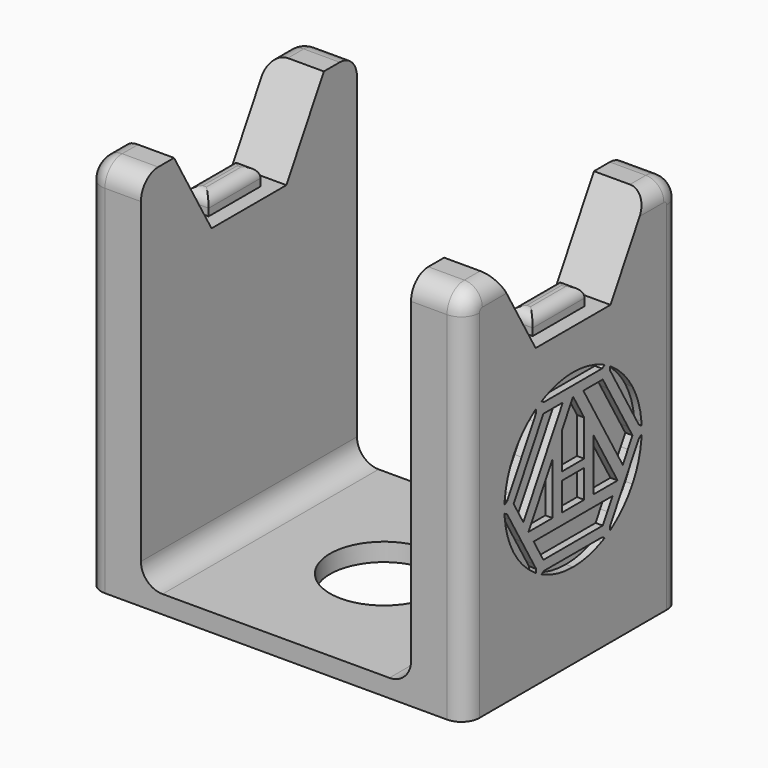
from build123d import *

# Parameters (mm, degrees)
F1_DEPTH  = 75
F3_DEPTH  = 122
F4_W      = 7
F4_H      = 18
F5_DEPTH  = 5
F6_R      = 3
F7_R      = 6
F8_R      = 5
F10_DEPTH = 2
F12_DEPTH = 2
F14_DEPTH = 25


with BuildPart() as f1:
    # F0 (on Front) → F1 (new body)
    with BuildSketch(Plane.XZ):
        Polygon((-52.5, -2.5), (52.5, -2.5), (52.5, 2.5), (37.5, 2.5), (0, 2.5), (-37.5, 2.5), (-52.5, 2.5), align=None)
        Polygon((37.5, 2.5), (52.5, 2.5), (52.5, 102.5), (37.5, 102.5), (37.5, 40), align=None)
        Polygon((-52.5, 102.5), (-52.5, 2.5), (-37.5, 2.5), (-37.5, 40), (-37.5, 102.5), align=None)
    extrude(amount=F1_DEPTH)

    # F2 (on face) → F3 (cut)
    with BuildSketch(Plane.YZ.offset(52.5)):
        Polygon((-24.5, 79.9833395016), (-11.5, 102.5), (-24.5, 125.0166604984), (-50.5, 125.0166604984), (-63.5, 102.5), (-50.5, 79.9833395016), align=None)
    extrude(amount=-F3_DEPTH, mode=Mode.SUBTRACT)

    # F4 (on face) → F5 (join)
    with BuildSketch(Plane.XY.offset(79.9833395016)):
        with Locations((45, -37.5)):
            Rectangle(F4_W, F4_H)
        with Locations((-45, -37.5)):
            Rectangle(F4_W, F4_H)
    extrude(amount=F5_DEPTH)

    # F6
    f6_edges = [f1.edges().sort_by_distance(p)[0] for p in [
        (-48.5, -37.5, 84.98334),
        (-45, -28.5, 84.98334),
        (-41.5, -37.5, 84.98334),
        (-45, -46.5, 84.98334),
        (41.5, -37.5, 84.98334),
        (45, -28.5, 84.98334),
        (48.5, -37.5, 84.98334),
        (45, -46.5, 84.98334),
    ]]
    fillet(f6_edges, radius=F6_R)

    # F7
    f7_edges = [f1.edges().sort_by_distance(p)[0] for p in [
        (-37.5, -37.5, 2.5),
        (37.5, -37.5, 2.5),
        (-45, -75, 102.5),
        (45, -75, 102.5),
        (45, 0, 102.5),
        (-45, 0, 102.5),
    ]]
    fillet(f7_edges, radius=F7_R)

    # F8
    f8_edges = [f1.edges().sort_by_distance(p)[0] for p in [
        (-52.5, -75, 47),
        (-52.5, 0, 47),
        (52.5, -75, 47),
        (52.5, 0, 47),
        (-52.5, -1.757359, 100.742641),
        (-52.5, -8.75, 102.5),
        (-52.5, -73.242641, 100.742641),
        (-52.5, -66.25, 102.5),
        (52.5, -1.757359, 100.742641),
        (52.5, -8.75, 102.5),
        (52.5, -73.242641, 100.742641),
        (52.5, -66.25, 102.5),
    ]]
    fillet(f8_edges, radius=F8_R)

    # F9 (on face) → F10 (cut)
    with BuildSketch(Plane.YZ.offset(52.5)):
        with BuildLine():
            Line((-19.6382260469, 34.6708395016), (-16.875, 33.0754901996))
            ThreePointArc((-16.875, 33.0754901996), (-14.8031482966, 37.7694346816), (-13.7847580184, 42.7982084409))
            Line((-13.7847580184, 42.7982084409), (-15.5264520939, 41.7926408975))
            Line((-15.5264520939, 41.7926408975), (-19.6382260469, 34.6708395016))
        make_face()
        with BuildLine():
            ThreePointArc((-23.75, 25.537903019), (-19.9041493137, 28.9342417505), (-16.875, 33.0754901996))
            Line((-16.875, 33.0754901996), (-19.6382260469, 34.6708395016))
            Line((-19.6382260469, 34.6708395016), (-23.75, 27.5490381057))
            Line((-23.75, 27.5490381057), (-23.75, 25.537903019))
        make_face()
        with BuildLine():
            ThreePointArc((-13.7847580184, 47.1684705623), (-14.8031482746, 52.1972442527), (-16.8749999276, 56.8911886783))
            ThreePointArc((-16.8749999276, 56.8911886783), (-19.9041492649, 61.0324371992), (-23.75, 64.4287759842))
            Line((-23.75, 64.4287759842), (-23.75, 62.4176408975))
            Line((-23.75, 62.4176408975), (-19.6382260214, 55.2958394574))
            Line((-19.6382260214, 55.2958394574), (-15.5264520939, 48.1740381057))
            Line((-15.5264520939, 48.1740381057), (-13.7847580184, 47.1684705623))
        make_face()
        with BuildLine():
            Line((-37.5, 65.6083395016), (-37.5, 68.7990381057))
            ThreePointArc((-37.5, 68.7990381057), (-42.6010010171, 68.2463420727), (-47.4652419816, 66.613907045))
            Line((-47.4652419816, 66.613907045), (-45.7235479061, 65.6083395016))
            Line((-45.7235479061, 65.6083395016), (-37.5, 65.6083395016))
        make_face()
        with BuildLine():
            ThreePointArc((-27.5347580184, 66.613907045), (-32.3989989829, 68.2463420727), (-37.5, 68.7990381057))
            Line((-37.5, 68.7990381057), (-37.5, 65.6083395016))
            Line((-37.5, 65.6083395016), (-29.2764520939, 65.6083395016))
            Line((-29.2764520939, 65.6083395016), (-27.5347580184, 66.613907045))
        make_face()
        with BuildLine():
            ThreePointArc((-47.4652419816, 23.3527719583), (-42.6010010171, 21.7203369305), (-37.5, 21.1676408975))
            ThreePointArc((-37.5, 21.1676408975), (-32.3989989829, 21.7203369305), (-27.5347580184, 23.3527719583))
            Line((-27.5347580184, 23.3527719583), (-29.2764520939, 24.3583395016))
            Line((-29.2764520939, 24.3583395016), (-37.5, 24.3583395016))
            Line((-37.5, 24.3583395016), (-45.7235479061, 24.3583395016))
            Line((-45.7235479061, 24.3583395016), (-47.4652419816, 23.3527719583))
        make_face()
        with BuildLine():
            ThreePointArc((-24.671075349, 24.9182904785), (-24.206927036, 25.2227294105), (-23.75, 25.537903019))
            Line((-23.75, 25.537903019), (-23.75, 27.5490381057))
            Line((-23.75, 27.5490381057), (-24.671075349, 25.9536888036))
            Line((-24.671075349, 25.9536888036), (-24.671075349, 24.9182904785))
        make_face()
        with BuildLine():
            Line((-15.5264520939, 41.7926408975), (-13.7847580184, 42.7982084409))
            ThreePointArc((-13.7847580184, 42.7982084409), (-13.7402731848, 43.351505666), (-13.7086954923, 43.9056893621))
            Line((-13.7086954923, 43.9056893621), (-14.6053767449, 43.3879901996))
            Line((-14.6053767449, 43.3879901996), (-15.5264520939, 41.7926408975))
        make_face()
        with BuildLine():
            ThreePointArc((-13.7086954923, 46.0609896411), (-13.7402731848, 46.6151733372), (-13.7847580184, 47.1684705623))
            Line((-13.7847580184, 47.1684705623), (-15.5264520939, 48.1740381057))
            Line((-15.5264520939, 48.1740381057), (-14.6053767449, 46.5786888036))
            Line((-14.6053767449, 46.5786888036), (-13.7086954923, 46.0609896411))
        make_face()
        with BuildLine():
            Line((-23.75, 62.4176408975), (-23.75, 64.4287759842))
            ThreePointArc((-23.75, 64.4287759842), (-24.206927036, 64.7439495927), (-24.671075349, 65.0483885247))
            Line((-24.671075349, 65.0483885247), (-24.671075349, 64.0129901996))
            Line((-24.671075349, 64.0129901996), (-23.75, 62.4176408975))
        make_face()
        with BuildLine():
            ThreePointArc((-26.5376201433, 66.1260386642), (-27.0333461488, 66.3757834284), (-27.5347580184, 66.613907045))
            Line((-27.5347580184, 66.613907045), (-29.2764520939, 65.6083395016))
            Line((-29.2764520939, 65.6083395016), (-27.4343013959, 65.6083395016))
            Line((-27.4343013959, 65.6083395016), (-26.5376201433, 66.1260386642))
        make_face()
        with BuildLine():
            Line((-45.7235479061, 65.6083395016), (-47.4652419816, 66.613907045))
            ThreePointArc((-47.4652419816, 66.613907045), (-47.9666538512, 66.3757834284), (-48.4623798567, 66.1260386642))
            Line((-48.4623798567, 66.1260386642), (-47.5656986041, 65.6083395016))
            Line((-47.5656986041, 65.6083395016), (-45.7235479061, 65.6083395016))
        make_face()
        with BuildLine():
            Line((-55.3617739531, 34.6708395016), (-58.125, 33.0754901996))
            ThreePointArc((-58.125, 33.0754901996), (-55.0958506863, 28.9342417505), (-51.25, 25.537903019))
            Line((-51.25, 25.537903019), (-51.25, 27.5490381057))
            Line((-51.25, 27.5490381057), (-55.3617739531, 34.6708395016))
        make_face()
        with BuildLine():
            ThreePointArc((-61.2152419816, 42.7982084409), (-60.1968517034, 37.7694346816), (-58.125, 33.0754901996))
            Line((-58.125, 33.0754901996), (-55.3617739531, 34.6708395016))
            Line((-55.3617739531, 34.6708395016), (-59.4735479061, 41.7926408975))
            Line((-59.4735479061, 41.7926408975), (-61.2152419816, 42.7982084409))
        make_face()
        with BuildLine():
            ThreePointArc((-48.4623798567, 23.840640339), (-47.9666538512, 23.5908955749), (-47.4652419816, 23.3527719583))
            Line((-47.4652419816, 23.3527719583), (-45.7235479061, 24.3583395016))
            Line((-45.7235479061, 24.3583395016), (-47.5656986041, 24.3583395016))
            Line((-47.5656986041, 24.3583395016), (-48.4623798567, 23.840640339))
        make_face()
        with BuildLine():
            Line((-29.2764520939, 24.3583395016), (-27.5347580184, 23.3527719583))
            ThreePointArc((-27.5347580184, 23.3527719583), (-27.0333461488, 23.5908955749), (-26.5376201433, 23.840640339))
            Line((-26.5376201433, 23.840640339), (-27.4343013959, 24.3583395016))
            Line((-27.4343013959, 24.3583395016), (-29.2764520939, 24.3583395016))
        make_face()
        Polygon((-30.3781986041, 27.1215655486), (-27.1875, 27.1215655486), (-25.592150698, 29.8847915955), align=None)
        Polygon((-18.470349302, 42.2201134547), (-16.875, 44.9833395016), (-18.470349302, 47.7465655486), align=None)
        with BuildLine():
            ThreePointArc((-51.25, 64.4287759842), (-55.0958506625, 61.0324372788), (-58.1249999646, 56.891188865))
            ThreePointArc((-58.1249999646, 56.891188865), (-60.1968516927, 52.1972443554), (-61.2152419816, 47.1684705623))
            Line((-61.2152419816, 47.1684705623), (-59.4735479061, 48.1740381057))
            Line((-59.4735479061, 48.1740381057), (-55.3617738149, 55.295839741))
            Line((-55.3617738149, 55.295839741), (-51.25, 62.4176408975))
            Line((-51.25, 62.4176408975), (-51.25, 64.4287759842))
        make_face()
        Polygon((-25.592150698, 60.0818874077), (-27.1875, 62.8451134547), (-30.3781986041, 62.8451134547), align=None)
        Polygon((-44.6218013959, 62.8451134547), (-47.8125, 62.8451134547), (-49.407849302, 60.0818874077), align=None)
        Polygon((-37.5, 46.0997003737), (-37.5, 62.8451134547), (-41.3671875, 56.1469482223), (-41.3671875, 46.0997003737), align=None)
        Polygon((-33.6328125, 56.1469482223), (-37.5, 62.8451134547), (-37.5, 46.0997003737), (-33.6328125, 46.0997003737), align=None)
        with BuildLine():
            ThreePointArc((-61.2913045077, 43.9056893621), (-61.2597268152, 43.351505666), (-61.2152419816, 42.7982084409))
            Line((-61.2152419816, 42.7982084409), (-59.4735479061, 41.7926408975))
            Line((-59.4735479061, 41.7926408975), (-60.3946232551, 43.3879901996))
            Line((-60.3946232551, 43.3879901996), (-61.2913045077, 43.9056893621))
        make_face()
        with BuildLine():
            Line((-51.25, 27.5490381057), (-51.25, 25.537903019))
            ThreePointArc((-51.25, 25.537903019), (-50.793072964, 25.2227294105), (-50.328924651, 24.9182904785))
            Line((-50.328924651, 24.9182904785), (-50.328924651, 25.9536888036))
            Line((-50.328924651, 25.9536888036), (-51.25, 27.5490381057))
        make_face()
        Polygon((-37.5, 27.1215655486), (-30.3781986041, 27.1215655486), (-25.592150698, 29.8847915955), (-23.811700349, 32.9686220603), (-51.188299651, 32.9686220603), (-49.407849302, 29.8847915955), (-44.6218013959, 27.1215655486), align=None)
        Polygon((-20.250799651, 39.1362829899), (-18.470349302, 42.2201134547), (-18.470349302, 47.7465655486), (-25.592150698, 60.0818874077), (-30.3781986041, 62.8451134547), (-33.939099302, 62.8451134547), align=None)
        with BuildLine():
            ThreePointArc((-50.328924651, 65.0483885247), (-50.793072964, 64.7439495927), (-51.25, 64.4287759842))
            Line((-51.25, 64.4287759842), (-51.25, 62.4176408975))
            Line((-51.25, 62.4176408975), (-50.328924651, 64.0129901996))
            Line((-50.328924651, 64.0129901996), (-50.328924651, 65.0483885247))
        make_face()
        with BuildLine():
            Line((-59.4735479061, 48.1740381057), (-61.2152419816, 47.1684705623))
            ThreePointArc((-61.2152419816, 47.1684705623), (-61.2597268152, 46.6151733372), (-61.2913045077, 46.0609896411))
            Line((-61.2913045077, 46.0609896411), (-60.3946232551, 46.5786888036))
            Line((-60.3946232551, 46.5786888036), (-59.4735479061, 48.1740381057))
        make_face()
        Polygon((-44.6218013959, 62.8451134547), (-49.407849302, 60.0818874077), (-56.529650698, 47.7465655486), (-56.529650698, 42.2201134547), (-54.749200349, 39.1362829899), (-41.060900698, 62.8451134547), align=None)
        Polygon((-56.529650698, 47.7465655486), (-58.125, 44.9833395016), (-56.529650698, 42.2201134547), align=None)
        Polygon((-49.407849302, 29.8847915955), (-47.8125, 27.1215655486), (-44.6218013959, 27.1215655486), align=None)
        Polygon((-45.234375, 49.4487829899), (-52.96875, 36.0524525251), (-44.6218013959, 36.0524525251), (-44.6218013959, 50.5097915955), align=None)
        Polygon((-29.765625, 49.4487829899), (-30.3781986041, 50.5097915955), (-30.3781986041, 36.0524525251), (-22.03125, 36.0524525251), align=None)
        Polygon((-41.3671875, 40.5178960133), (-41.3671875, 36.0524525251), (-33.6328125, 36.0524525251), (-33.6328125, 43.8669786295), (-37.5, 43.8669786295), (-41.3671875, 43.8669786295), (-41.3671875, 42.7506177575), align=None)
    extrude(amount=-F10_DEPTH, mode=Mode.SUBTRACT)

    # F11 (on face) → F12 (cut)
    with BuildSketch(Plane(origin=(-52.5, 0, 0), x_dir=(0, -1, 0), z_dir=(-1, 0, 0))):
        with BuildLine():
            Line((55.3617739531, 34.6708395016), (58.125, 33.0754901996))
            ThreePointArc((58.125, 33.0754901996), (60.1968517034, 37.7694346816), (61.2152419816, 42.7982084409))
            Line((61.2152419816, 42.7982084409), (59.4735479061, 41.7926408975))
            Line((59.4735479061, 41.7926408975), (55.3617739531, 34.6708395016))
        make_face()
        with BuildLine():
            ThreePointArc((51.25, 25.537903019), (55.0958506863, 28.9342417505), (58.125, 33.0754901996))
            Line((58.125, 33.0754901996), (55.3617739531, 34.6708395016))
            Line((55.3617739531, 34.6708395016), (51.25, 27.5490381057))
            Line((51.25, 27.5490381057), (51.25, 25.537903019))
        make_face()
        with BuildLine():
            ThreePointArc((61.2152419816, 47.1684705623), (60.1968520672, 52.197243177), (58.1250012011, 56.8911867233))
            ThreePointArc((58.1250012011, 56.8911867233), (55.0958514957, 61.0324363653), (51.25, 64.4287759842))
            Line((51.25, 64.4287759842), (51.25, 62.4176408975))
            Line((51.25, 62.4176408975), (55.3617761034, 55.2958357771))
            Line((55.3617761034, 55.2958357771), (59.4735479061, 48.1740381057))
            Line((59.4735479061, 48.1740381057), (61.2152419816, 47.1684705623))
        make_face()
        with BuildLine():
            Line((37.5, 65.6083395016), (37.5, 68.7990381057))
            ThreePointArc((37.5, 68.7990381057), (32.3989989829, 68.2463420727), (27.5347580184, 66.613907045))
            Line((27.5347580184, 66.613907045), (29.2764520939, 65.6083395016))
            Line((29.2764520939, 65.6083395016), (37.5, 65.6083395016))
        make_face()
        with BuildLine():
            ThreePointArc((47.4652419816, 66.613907045), (42.6010010171, 68.2463420727), (37.5, 68.7990381057))
            Line((37.5, 68.7990381057), (37.5, 65.6083395016))
            Line((37.5, 65.6083395016), (45.7235479061, 65.6083395016))
            Line((45.7235479061, 65.6083395016), (47.4652419816, 66.613907045))
        make_face()
        with BuildLine():
            ThreePointArc((27.5347580184, 23.3527719583), (32.3989989829, 21.7203369305), (37.5, 21.1676408975))
            ThreePointArc((37.5, 21.1676408975), (42.6010010171, 21.7203369305), (47.4652419816, 23.3527719583))
            Line((47.4652419816, 23.3527719583), (45.7235479061, 24.3583395016))
            Line((45.7235479061, 24.3583395016), (37.5, 24.3583395016))
            Line((37.5, 24.3583395016), (29.2764520939, 24.3583395016))
            Line((29.2764520939, 24.3583395016), (27.5347580184, 23.3527719583))
        make_face()
        with BuildLine():
            ThreePointArc((50.328924651, 24.9182904785), (50.793072964, 25.2227294105), (51.25, 25.537903019))
            Line((51.25, 25.537903019), (51.25, 27.5490381057))
            Line((51.25, 27.5490381057), (50.328924651, 25.9536888036))
            Line((50.328924651, 25.9536888036), (50.328924651, 24.9182904785))
        make_face()
        with BuildLine():
            Line((59.4735479061, 41.7926408975), (61.2152419816, 42.7982084409))
            ThreePointArc((61.2152419816, 42.7982084409), (61.2597268152, 43.351505666), (61.2913045077, 43.9056893621))
            Line((61.2913045077, 43.9056893621), (60.3946232551, 43.3879901996))
            Line((60.3946232551, 43.3879901996), (59.4735479061, 41.7926408975))
        make_face()
        with BuildLine():
            ThreePointArc((61.2913045077, 46.0609896411), (61.2597268152, 46.6151733372), (61.2152419816, 47.1684705623))
            Line((61.2152419816, 47.1684705623), (59.4735479061, 48.1740381057))
            Line((59.4735479061, 48.1740381057), (60.3946232551, 46.5786888036))
            Line((60.3946232551, 46.5786888036), (61.2913045077, 46.0609896411))
        make_face()
        with BuildLine():
            Line((51.25, 62.4176408975), (51.25, 64.4287759842))
            ThreePointArc((51.25, 64.4287759842), (50.793072964, 64.7439495927), (50.328924651, 65.0483885247))
            Line((50.328924651, 65.0483885247), (50.328924651, 64.0129901996))
            Line((50.328924651, 64.0129901996), (51.25, 62.4176408975))
        make_face()
        with BuildLine():
            ThreePointArc((48.4623798567, 66.1260386642), (47.9666538512, 66.3757834284), (47.4652419816, 66.613907045))
            Line((47.4652419816, 66.613907045), (45.7235479061, 65.6083395016))
            Line((45.7235479061, 65.6083395016), (47.5656986041, 65.6083395016))
            Line((47.5656986041, 65.6083395016), (48.4623798567, 66.1260386642))
        make_face()
        with BuildLine():
            Line((29.2764520939, 65.6083395016), (27.5347580184, 66.613907045))
            ThreePointArc((27.5347580184, 66.613907045), (27.0333461488, 66.3757834284), (26.5376201433, 66.1260386642))
            Line((26.5376201433, 66.1260386642), (27.4343013959, 65.6083395016))
            Line((27.4343013959, 65.6083395016), (29.2764520939, 65.6083395016))
        make_face()
        with BuildLine():
            Line((19.6382260469, 34.6708395016), (16.875, 33.0754901996))
            ThreePointArc((16.875, 33.0754901996), (19.9041493137, 28.9342417505), (23.75, 25.537903019))
            Line((23.75, 25.537903019), (23.75, 27.5490381057))
            Line((23.75, 27.5490381057), (19.6382260469, 34.6708395016))
        make_face()
        with BuildLine():
            ThreePointArc((13.7847580184, 42.7982084409), (14.8031482966, 37.7694346816), (16.875, 33.0754901996))
            Line((16.875, 33.0754901996), (19.6382260469, 34.6708395016))
            Line((19.6382260469, 34.6708395016), (15.5264520939, 41.7926408975))
            Line((15.5264520939, 41.7926408975), (13.7847580184, 42.7982084409))
        make_face()
        with BuildLine():
            ThreePointArc((26.5376201433, 23.840640339), (27.0333461488, 23.5908955749), (27.5347580184, 23.3527719583))
            Line((27.5347580184, 23.3527719583), (29.2764520939, 24.3583395016))
            Line((29.2764520939, 24.3583395016), (27.4343013959, 24.3583395016))
            Line((27.4343013959, 24.3583395016), (26.5376201433, 23.840640339))
        make_face()
        with BuildLine():
            Line((45.7235479061, 24.3583395016), (47.4652419816, 23.3527719583))
            ThreePointArc((47.4652419816, 23.3527719583), (47.9666538512, 23.5908955749), (48.4623798567, 23.840640339))
            Line((48.4623798567, 23.840640339), (47.5656986041, 24.3583395016))
            Line((47.5656986041, 24.3583395016), (45.7235479061, 24.3583395016))
        make_face()
        Polygon((44.6218013959, 27.1215655486), (47.8125, 27.1215655486), (49.407849302, 29.8847915955), align=None)
        Polygon((56.529650698, 42.2201134547), (58.125, 44.9833395016), (56.529650698, 47.7465655486), align=None)
        with BuildLine():
            ThreePointArc((23.75, 64.4287759842), (19.9041485043, 61.0324363653), (16.8749987989, 56.8911867233))
            ThreePointArc((16.8749987989, 56.8911867233), (14.8031479328, 52.197243177), (13.7847580184, 47.1684705623))
            Line((13.7847580184, 47.1684705623), (15.5264520939, 48.1740381057))
            Line((15.5264520939, 48.1740381057), (19.6382240004, 55.2958359568))
            Line((19.6382240004, 55.2958359568), (23.75, 62.4176408975))
            Line((23.75, 62.4176408975), (23.75, 64.4287759842))
        make_face()
        Polygon((49.407849302, 60.0818874077), (47.8125, 62.8451134547), (44.6218013959, 62.8451134547), align=None)
        Polygon((30.3781986041, 62.8451134547), (27.1875, 62.8451134547), (25.592150698, 60.0818874077), align=None)
        Polygon((37.5, 46.0997003737), (37.5, 62.8451134547), (33.6328125, 56.1469482223), (33.6328125, 46.0997003737), align=None)
        Polygon((41.3671875, 56.1469482223), (37.5, 62.8451134547), (37.5, 46.0997003737), (41.3671875, 46.0997003737), align=None)
        with BuildLine():
            ThreePointArc((13.7086954923, 43.9056893621), (13.7402731848, 43.351505666), (13.7847580184, 42.7982084409))
            Line((13.7847580184, 42.7982084409), (15.5264520939, 41.7926408975))
            Line((15.5264520939, 41.7926408975), (14.6053767449, 43.3879901996))
            Line((14.6053767449, 43.3879901996), (13.7086954923, 43.9056893621))
        make_face()
        with BuildLine():
            Line((23.75, 27.5490381057), (23.75, 25.537903019))
            ThreePointArc((23.75, 25.537903019), (24.206927036, 25.2227294105), (24.671075349, 24.9182904785))
            Line((24.671075349, 24.9182904785), (24.671075349, 25.9536888036))
            Line((24.671075349, 25.9536888036), (23.75, 27.5490381057))
        make_face()
        Polygon((37.5, 27.1215655486), (44.6218013959, 27.1215655486), (49.407849302, 29.8847915955), (51.188299651, 32.9686220603), (23.811700349, 32.9686220603), (25.592150698, 29.8847915955), (30.3781986041, 27.1215655486), align=None)
        Polygon((54.749200349, 39.1362829899), (56.529650698, 42.2201134547), (56.529650698, 47.7465655486), (49.407849302, 60.0818874077), (44.6218013959, 62.8451134547), (41.060900698, 62.8451134547), align=None)
        with BuildLine():
            ThreePointArc((24.671075349, 65.0483885247), (24.206927036, 64.7439495927), (23.75, 64.4287759842))
            Line((23.75, 64.4287759842), (23.75, 62.4176408975))
            Line((23.75, 62.4176408975), (24.671075349, 64.0129901996))
            Line((24.671075349, 64.0129901996), (24.671075349, 65.0483885247))
        make_face()
        with BuildLine():
            Line((15.5264520939, 48.1740381057), (13.7847580184, 47.1684705623))
            ThreePointArc((13.7847580184, 47.1684705623), (13.7402731848, 46.6151733372), (13.7086954923, 46.0609896411))
            Line((13.7086954923, 46.0609896411), (14.6053767449, 46.5786888036))
            Line((14.6053767449, 46.5786888036), (15.5264520939, 48.1740381057))
        make_face()
        Polygon((30.3781986041, 62.8451134547), (25.592150698, 60.0818874077), (18.470349302, 47.7465655486), (18.470349302, 42.2201134547), (20.250799651, 39.1362829899), (33.939099302, 62.8451134547), align=None)
        Polygon((18.470349302, 47.7465655486), (16.875, 44.9833395016), (18.470349302, 42.2201134547), align=None)
        Polygon((25.592150698, 29.8847915955), (27.1875, 27.1215655486), (30.3781986041, 27.1215655486), align=None)
        Polygon((29.765625, 49.4487829899), (22.03125, 36.0524525251), (30.3781986041, 36.0524525251), (30.3781986041, 50.5097915955), align=None)
        Polygon((45.234375, 49.4487829899), (44.6218013959, 50.5097915955), (44.6218013959, 36.0524525251), (52.96875, 36.0524525251), align=None)
        Polygon((33.6328125, 40.5178960133), (33.6328125, 36.0524525251), (41.3671875, 36.0524525251), (41.3671875, 43.8669786295), (37.5, 43.8669786295), (33.6328125, 43.8669786295), (33.6328125, 42.7506177575), align=None)
    extrude(amount=-F12_DEPTH, mode=Mode.SUBTRACT)

    # F13 (on face) → F14 (cut)
    with BuildSketch(Plane.XY.offset(2.5)):
        with BuildLine():
            ThreePointArc((0, -22.5), (-10.6066017178, -48.1066017178), (15, -37.5))
            ThreePointArc((15, -37.5), (10.6066017178, -26.8933982822), (0, -22.5))
        make_face()
    extrude(amount=-F14_DEPTH, mode=Mode.SUBTRACT)


solid = f1.part
